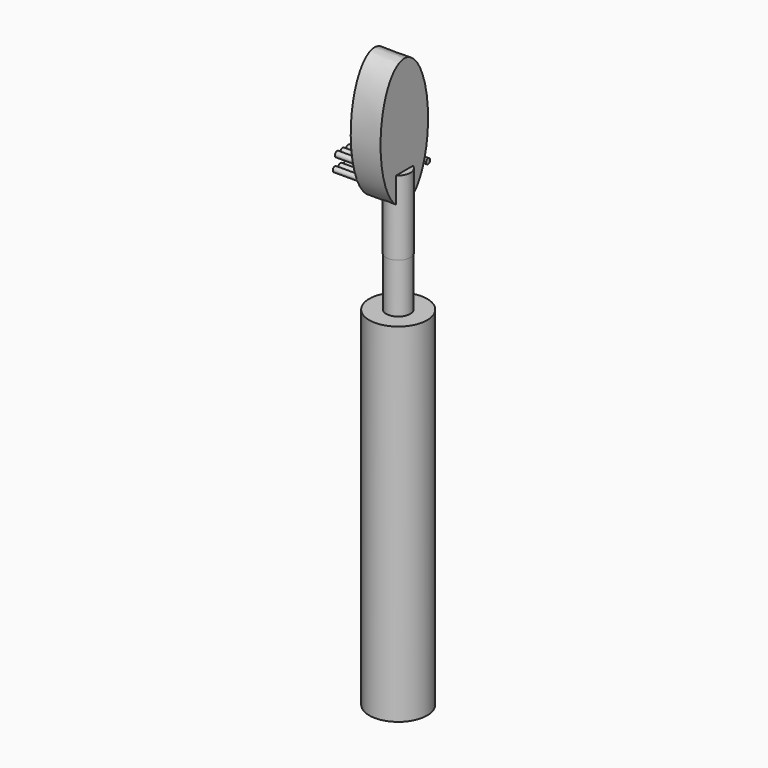
from build123d import *

# Parameters (mm, degrees)
F1_DEPTH = 15.24
F2_R     = 6.1393215521
F3_DEPTH = 203.2
F4_R     = 1.4250163951
F4_R_2   = 1.3335584615
F5_DEPTH = 12.7
F4_R_3   = 1.3335599772
F6_R     = 14.7875106542
F7_DEPTH = 177.8
F8_R     = 6.2626412316
F9_DEPTH = 38.1


with BuildPart() as f1:
    # F0 (on Right) → F1 (new body)
    with BuildSketch(Plane.YZ):
        with BuildLine():
            add(Edge.make_bspline(
                [(-23.3988817781, 22.8842264041), (2.8830545158, 22.8842264041), (-10.2579136311, 72.2143235616), (-23.3988817781, 121.5444207191), (-36.5398499251, 72.2143235616), (-49.6808180721, 22.8842264041), (-23.3988817781, 22.8842264041)],
                knots=[0, 0, 0, 2.0943951024, 2.0943951024, 4.1887902048, 4.1887902048, 6.2831853072, 6.2831853072, 6.2831853072], degree=2, weights=[1, 0.5, 1, 0.5, 1, 0.5, 1]))
        make_face()
    extrude(amount=F1_DEPTH)

    # F4 (on face) → F5 (join)
    with BuildSketch(Plane(origin=(0, 0, 0), x_dir=(0, -1, 0), z_dir=(-1, 0, 0))):
        with Locations((13.6097577012, 39.78548944)):
            Circle(F4_R)
        with Locations((17.1657577012, 39.78548944)):
            Circle(F4_R)
        with Locations((20.7217577012, 39.78548944)):
            Circle(F4_R)
        with Locations((24.2777577012, 39.78548944)):
            Circle(F4_R)
        with Locations((27.8337577012, 39.78548944)):
            Circle(F4_R)
        with Locations((31.3897577012, 39.78548944)):
            Circle(F4_R)
        with Locations((11.4777320996, 33.5845500231)):
            Circle(F4_R_2)
        with Locations((15.0337320996, 33.5845500231)):
            Circle(F4_R_2)
        with Locations((18.5897320996, 33.5845500231)):
            Circle(F4_R_2)
        with Locations((22.1457320996, 33.5845500231)):
            Circle(F4_R_2)
        with Locations((25.7017320996, 33.5845500231)):
            Circle(F4_R_2)
        with Locations((29.2577320996, 33.5845500231)):
            Circle(F4_R_2)
        with Locations((32.8137320996, 33.5845500231)):
            Circle(F4_R_2)
    extrude(amount=F5_DEPTH)


with BuildPart() as f3:
    # F2 (on Top) → F3 (new body)
    with BuildSketch(Plane.XY):
        with Locations((11.9830649346, -23.2287105173)):
            Circle(F2_R)
    extrude(amount=-F3_DEPTH)


with BuildPart() as f5:
    # F4 (on face) → F5, piece 2 (new body)
    with BuildSketch(Plane(origin=(0, 0, 0), x_dir=(0, -1, 0), z_dir=(-1, 0, 0))):
        with Locations((9.205583483, 28.4687820822)):
            Circle(F4_R_3)
    extrude(amount=F5_DEPTH)


with BuildPart() as f5b:
    # F4 (on face) → F5, piece 3 (new body)
    with BuildSketch(Plane(origin=(0, 0, 0), x_dir=(0, -1, 0), z_dir=(-1, 0, 0))):
        with Locations((-10.792426765, 23.5080346465)):
            Circle(F4_R_2)
    extrude(amount=F5_DEPTH)


with BuildPart() as f7:
    # F6 (on face) → F7 (new body)
    with BuildSketch(Plane(origin=(0, 0, -203.2), x_dir=(1, 0, 0), z_dir=(0, 0, -1))):
        with Locations((11.9830649346, 23.2287105173)):
            Circle(F6_R)
    extrude(amount=-F7_DEPTH)


with BuildPart() as f9:
    # F8 (on face) → F9 (new body)
    with BuildSketch(Plane.XY):
        with Locations((11.9830649346, -23.2287105173)):
            Circle(F8_R)
    extrude(amount=F9_DEPTH)


solid = Compound([f1.part, f3.part, f5.part, f5b.part, f7.part, f9.part])
